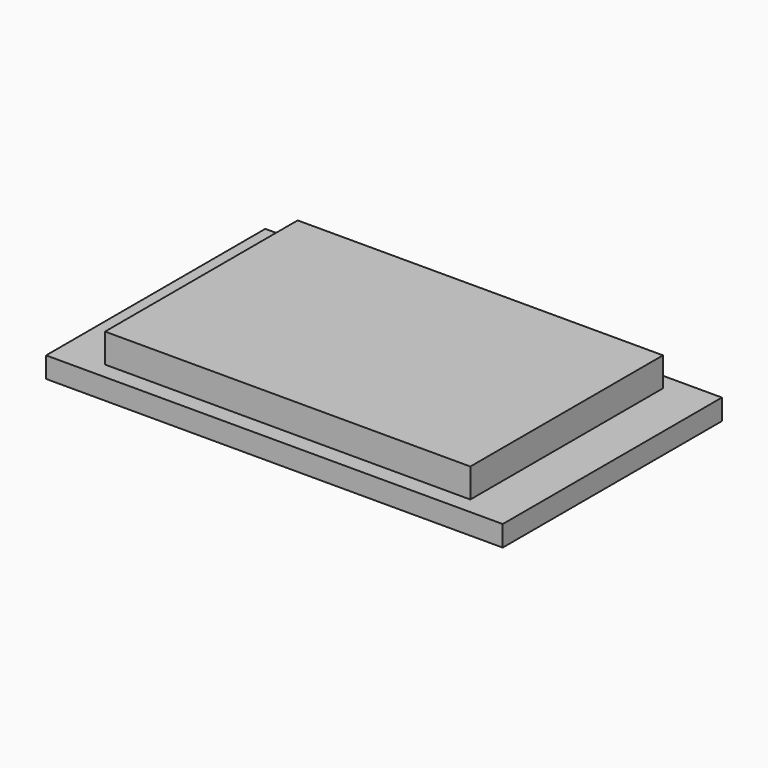
from build123d import *

# Parameters (mm, degrees)
F0_W         = 110
F0_H         = 66
F1_DEPTH     = 5
F2_W         = 88
F2_H         = 58
F3_DEPTH     = 7
F4_TEXT_SIZE = 36.2098630932
F5_DEPTH     = 6


# Not quite as in the source:
# - Text() gives the source's letters only with a copy of the font that has no kerning and outlines rounded to 1/6400 em; it was checked with that copy


with BuildPart() as f1:
    # F0 (on Top) → F1 (new body)
    with BuildSketch(Plane.XY):
        Rectangle(F0_W, F0_H)
    extrude(amount=F1_DEPTH)

    # F4 (on face) → F5 (cut)
    with BuildSketch(Plane(origin=(0, 0, 0), x_dir=(1, 0, 0), z_dir=(0, 0, -1))):
        with Locations((-28.6256745458, -14.6801620722)):
            Text('S.C.', F4_TEXT_SIZE, font='Open Sans', font_style=FontStyle.ITALIC, text_align=(TextAlign.LEFT, TextAlign.BOTTOM))
    extrude(amount=-F5_DEPTH, mode=Mode.SUBTRACT)


with BuildPart() as f3:
    # F2 (on face) → F3 (new body)
    with BuildSketch(Plane.XY.offset(5)):
        Rectangle(F2_W, F2_H)
    extrude(amount=F3_DEPTH)


solid = Compound([f1.part, f3.part])
